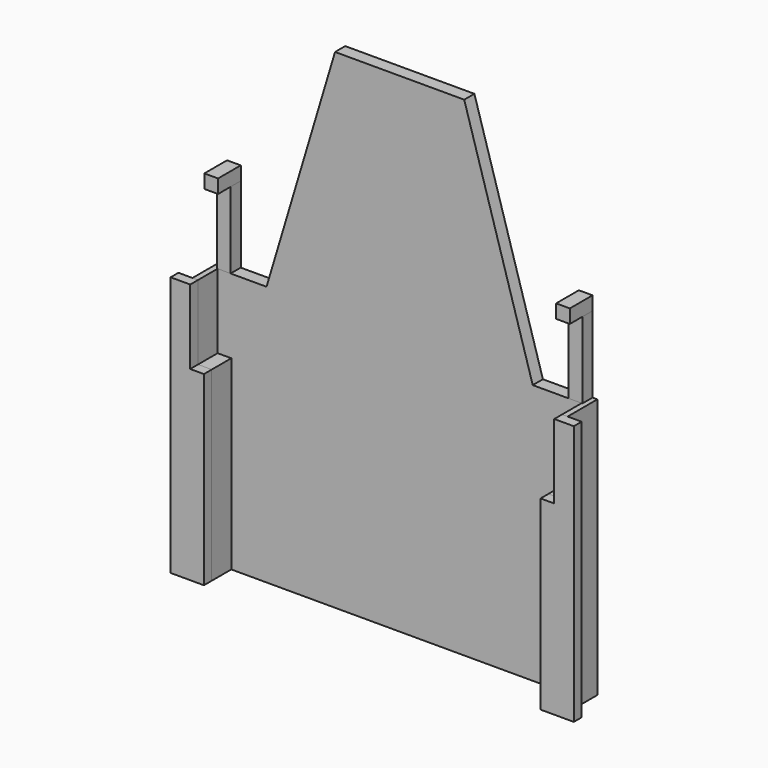
from build123d import *

# Parameters (mm, degrees)
F0_W     = 3.5839973688
F0_H     = 66.5
F1_DEPTH = 2.5
F2_DEPTH = 9.5
F4_DEPTH = 3.25
F5_W     = 3.5
F5_H     = 19.5
F6_DEPTH = 3.25
F5_H_2   = 3.5
F7_DEPTH = 7.25


# Not quite as in the source:
# - a feature names something its author has since deleted; it is built from what else it names


with BuildPart() as f1:
    # F0 (on Front) → F1 (new body)
    with BuildSketch(Plane.XZ):
        with Locations((-24.1530238986, -11.5398805141)):
            Rectangle(F0_W, F0_H)
        Polygon((-20.945022583, 21.7101194859), (-22.3610252142, 21.7101194859), (-22.3610252142, -44.7898805141), (-17.445022583, -44.7898805141), (-17.445022583, 2.7101194859), (-20.945022583, 2.7101194859), align=None)
    extrude(amount=F1_DEPTH)


with BuildPart() as f1b:
    # F0 (on Front) → F1, piece 2 (new body)
    with BuildSketch(Plane.XZ):
        with Locations((75.2629787326, -11.5398805141)):
            Rectangle(F0_W, F0_H)
        Polygon((68.554977417, 2.7101194859), (68.554977417, -44.7898805141), (73.4709800482, -44.7898805141), (73.4709800482, 21.7101194859), (72.054977417, 21.7101194859), (72.054977417, 2.7101194859), align=None)
    extrude(amount=F1_DEPTH)


with BuildPart() as f2:
    # F0 (on Front) → F2 (new body)
    with BuildSketch(Plane.XZ):
        Polygon((-20.945022583, 21.7101194859), (-22.3610252142, 21.7101194859), (-22.3610252142, -44.7898805141), (-17.445022583, -44.7898805141), (-17.445022583, 2.7101194859), (-20.945022583, 2.7101194859), align=None)
    extrude(amount=-F2_DEPTH)


with BuildPart() as f2b:
    # F0 (on Front) → F2, piece 2 (new body)
    with BuildSketch(Plane.XZ):
        Polygon((68.554977417, 2.7101194859), (68.554977417, -44.7898805141), (73.4709800482, -44.7898805141), (73.4709800482, 21.7101194859), (72.054977417, 21.7101194859), (72.054977417, 2.7101194859), align=None)
    extrude(amount=-F2_DEPTH)

    # F3 (on face) → F4 (join)
    with BuildSketch(Plane(origin=(0, 9.5, 0), x_dir=(-1, 0, 0), z_dir=(0, 1, 0))):
        Polygon((20.945022583, 2.7101194859), (20.945022583, 21.7101194859), (8.4450252142, 21.7101194859), (-25.5549747858, 21.7101194859), (-25.5549747858, -44.7898805141), (17.445022583, -44.7898805141), (17.445022583, 2.7101194859), align=None)
        Polygon((-25.5549747858, 21.7101194859), (8.4450252142, 21.7101194859), (-9.0549747858, 80.2101194859), (-25.5549747858, 80.2101194859), align=None)
        Polygon((-59.5549747858, 21.7101194859), (-25.5549747858, 21.7101194859), (-25.5549747858, 80.2101194859), (-42.0549747858, 80.2101194859), align=None)
        Polygon((-73.4709747858, -44.7898805141), (-25.5549747858, -44.7898805141), (-25.5549747858, 21.7101194859), (-59.5549747858, 21.7101194859), (-73.4709747858, 21.7101194859), align=None)
    extrude(amount=-F4_DEPTH)


with BuildPart() as f6:
    # F5 (on face) → F6 (new body)
    with BuildSketch(Plane(origin=(0, 9.5, 0), x_dir=(-1, 0, 0), z_dir=(0, 1, 0))):
        with Locations((-70.4882739186, 31.4602952302)):
            Rectangle(F5_W, F5_H)
    extrude(amount=-F6_DEPTH)


with BuildPart() as f6b:
    # F5 (on face) → F6, piece 2 (new body)
    with BuildSketch(Plane(origin=(0, 9.5, 0), x_dir=(-1, 0, 0), z_dir=(0, 1, 0))):
        with Locations((19.378324347, 31.4602952302)):
            Rectangle(F5_W, F5_H)
    extrude(amount=-F6_DEPTH)


with BuildPart() as f7:
    # F5 (on face) → F7 (new body)
    with BuildSketch(Plane(origin=(0, 9.5, 0), x_dir=(-1, 0, 0), z_dir=(0, 1, 0))):
        with Locations((-70.4882739186, 42.9602952302)):
            Rectangle(F5_W, F5_H_2)
    extrude(amount=-F7_DEPTH)


with BuildPart() as f7b:
    # F5 (on face) → F7, piece 2 (new body)
    with BuildSketch(Plane(origin=(0, 9.5, 0), x_dir=(-1, 0, 0), z_dir=(0, 1, 0))):
        with Locations((19.378324347, 42.9602952302)):
            Rectangle(F5_W, F5_H_2)
    extrude(amount=-F7_DEPTH)


solid = Compound([f1.part, f1b.part, f2.part, f2b.part, f6.part, f6b.part, f7.part, f7b.part])
